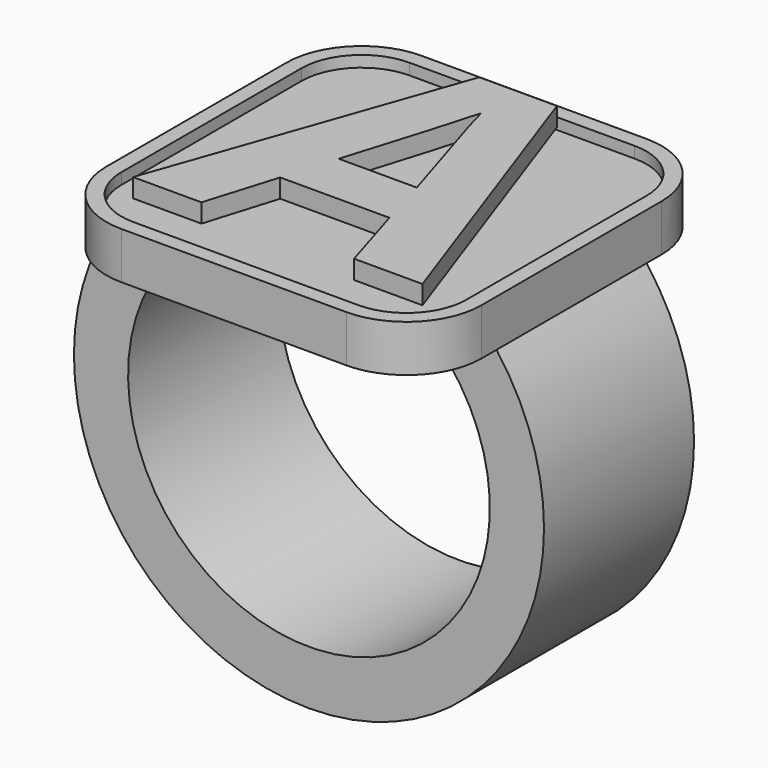
from build123d import *

# Parameters (mm, degrees)
F0_W          = 25.4
F0_H          = 25.4
F1_DEPTH      = 3.175
F3_W          = 5.08
F3_H          = 12.7
F6_DEPTH      = 6.35
F7_R          = 5.08
F10_DEPTH     = 0.762
F11_TEXT_SIZE = 28.4028821625
F12_DEPTH     = 1.27


# Not quite as in the source:
# - Text() gives the source's letters only with a copy of the font that has no kerning and outlines rounded to 1/6400 em; it was checked with that copy


with BuildPart() as f1:
    # F0 (on Top) → F1 (new body)
    with BuildSketch(Plane.XY):
        Rectangle(F0_W, F0_H)
    extrude(amount=F1_DEPTH)

    # F4: sweep along a path in F2
    with BuildLine(Plane.XZ) as f4_path:
        ThreePointArc((-10.16, 0), (0, -23.5582897328), (10.16, 0))
    # F3 (on face) → F4 (sweep)
    with BuildSketch(Plane(origin=(0, 0, 0), x_dir=(1, 0, 0), z_dir=(0, 0, -1))):
        with Locations((10.16, 0)):
            Rectangle(F3_W, F3_H)
    sweep(path=f4_path.line)

    # F5 (on Front) → F6 (join, symmetric)
    with BuildSketch(Plane.XZ):
        with BuildLine():
            ThreePointArc((-10.0130578512, -2.535746045), (-8.9072265211, -1.1822790439), (-7.62, 0))
            Line((-7.62, 0), (-10.16, 0))
            Line((-10.16, 0), (-10.0130578512, -2.535746045))
        make_face()
    extrude(amount=F6_DEPTH, both=True)

    # F7
    f7_edges = [f1.edges().sort_by_distance(p)[0] for p in [
        (12.7, -12.7, 1.5875),
        (-12.7, -12.7, 1.5875),
        (12.7, 12.7, 1.5875),
        (-12.7, 12.7, 1.5875),
    ]]
    fillet(f7_edges, radius=F7_R)

    # F9 (on face) → F10 (cut)
    with BuildSketch(Plane.XY.offset(3.175)):
        with BuildLine():
            ThreePointArc((11.6839997276, 7.62), (10.4936817661, 10.4936817661), (7.62, 11.6839997276))
            Line((7.62, 11.6839997276), (-7.62, 11.6839997276))
            ThreePointArc((-7.62, 11.6839997276), (-10.4936817661, 10.4936817661), (-11.6839997276, 7.62))
            Line((-11.6839997276, 7.62), (-11.6839997276, -7.62))
            ThreePointArc((-11.6839997276, -7.62), (-10.4936817661, -10.4936817661), (-7.62, -11.6839997276))
            Line((-7.62, -11.6839997276), (7.62, -11.6839997276))
            ThreePointArc((7.62, -11.6839997276), (10.4936817661, -10.4936817661), (11.6839997276, -7.62))
            Line((11.6839997276, -7.62), (11.6839997276, 7.62))
        make_face()
    extrude(amount=-F10_DEPTH, mode=Mode.SUBTRACT)


with BuildPart() as f12:
    # F11 (on face) → F12 (new body)
    with BuildSketch(Plane.XY.offset(3.175)):
        with Locations((-9.3301944435, -9.5796789974)):
            Text('A', F11_TEXT_SIZE, font='Open Sans', font_style=FontStyle.BOLD, text_align=(TextAlign.LEFT, TextAlign.BOTTOM))
    extrude(amount=F12_DEPTH)


solid = Compound([f1.part, f12.part])
